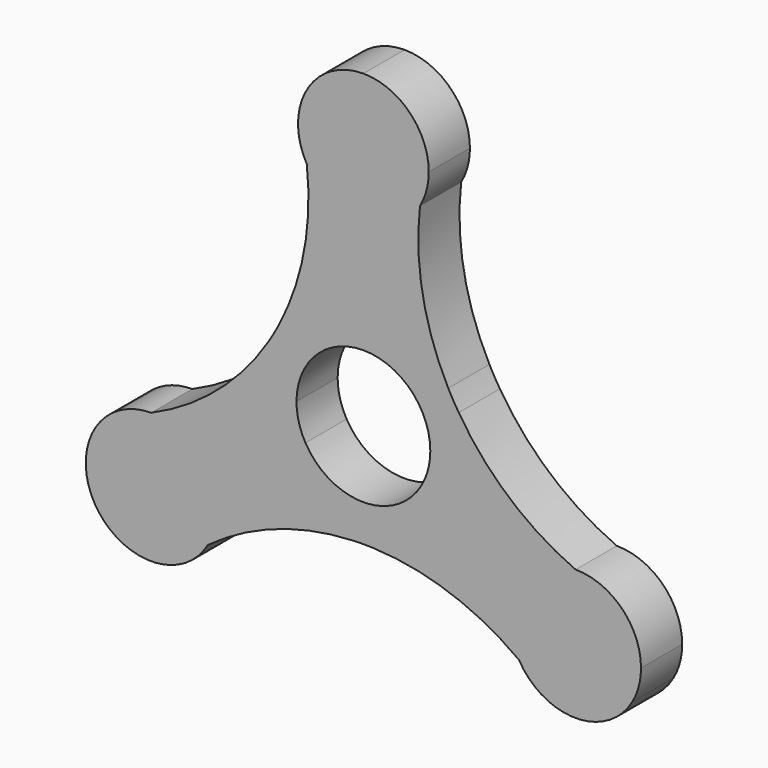
from build123d import *

# Parameters (mm, degrees)
F1_DEPTH = 5


# Not quite as in the source:
# - a feature names something its author has since deleted; it is built from what else it names


with BuildPart() as f1:
    # F0 (on Front) → F1 (new body)
    with BuildSketch(Plane.XZ):
        with BuildLine():
            ThreePointArc((-6.5, 0), (-4.5961940777, 4.5961940777), (0, 6.5))
            Line((0, 6.5), (0, 10.16))
            ThreePointArc((0, 10.16), (-4.6323577324, 9.0425030738), (-8.2456907547, 5.9358389447))
            ThreePointArc((-8.2456907547, 5.9358389447), (-8.7368966018, 5.0442496049), (-9.2634326962, 4.173058193))
            ThreePointArc((-9.2634326962, 4.173058193), (-9.9333296581, 2.1341419594), (-10.16, 0))
            Line((-10.16, 0), (-6.5, 0))
        make_face()
        with BuildLine():
            ThreePointArc((-5.6291651246, -3.25), (-6.2785178709, -1.6823237932), (-6.5, 0))
            Line((-6.5, 0), (-10.16, 0))
            ThreePointArc((-10.16, 0), (-9.8138063951, -2.6296014982), (-8.7988181024, -5.08))
            Line((-8.7988181024, -5.08), (-5.6291651246, -3.25))
        make_face()
        with BuildLine():
            ThreePointArc((-1.0177419415, -10.1088971377), (-0.508973166, -10.0935992038), (0, -10.0884992098))
            Line((0, -10.0884992098), (0, -6.5))
            ThreePointArc((0, -6.5), (-3.25, -5.6291651246), (-5.6291651246, -3.25))
            Line((-5.6291651246, -3.25), (-8.7988181024, -5.08))
            ThreePointArc((-8.7988181024, -5.08), (-5.5148585095, -8.5329910126), (-1.0177419415, -10.1088971377))
        make_face()
        with BuildLine():
            ThreePointArc((1.0177419415, -10.1088971377), (5.5148585095, -8.5329910126), (8.7988181024, -5.08))
            Line((8.7988181024, -5.08), (5.6291651246, -3.25))
            ThreePointArc((5.6291651246, -3.25), (3.25, -5.6291651246), (0, -6.5))
            Line((0, -6.5), (0, -10.0884992098))
            ThreePointArc((0, -10.0884992098), (0.508973166, -10.0935992038), (1.0177419415, -10.1088971377))
        make_face()
        with BuildLine():
            ThreePointArc((8.7988181024, -5.08), (9.8138063951, -2.6296014982), (10.16, 0))
            Line((10.16, 0), (6.5, 0))
            ThreePointArc((6.5, 0), (6.2785178709, -1.6823237932), (5.6291651246, -3.25))
            Line((5.6291651246, -3.25), (8.7988181024, -5.08))
        make_face()
        with BuildLine():
            Line((6.5, 0), (10.16, 0))
            ThreePointArc((10.16, 0), (9.9333296581, 2.1341419594), (9.2634326962, 4.173058193))
            ThreePointArc((9.2634326962, 4.173058193), (8.7368966018, 5.0442496049), (8.2456907547, 5.9358389447))
            ThreePointArc((8.2456907547, 5.9358389447), (4.6323577324, 9.0425030738), (0, 10.16))
            Line((0, 10.16), (0, 6.5))
            ThreePointArc((0, 6.5), (4.5961940777, 4.5961940777), (6.5, 0))
        make_face()
        with BuildLine():
            ThreePointArc((-8.2456907547, 5.9358389447), (-4.6323577324, 9.0425030738), (0, 10.16))
            Line((0, 10.16), (0, 15.875))
            Line((0, 15.875), (0, 17.4625))
            ThreePointArc((0, 17.4625), (-3.175, 18.313238686), (-5.499261314, 20.6375))
            ThreePointArc((-5.499261314, 20.6375), (-5.7658770412, 13.0799448007), (-8.2456907547, 5.9358389447))
        make_face()
        with BuildLine():
            Line((-5.499261314, 20.6375), (0, 23.8125))
            Line((0, 23.8125), (0, 30.1625))
            ThreePointArc((0, 30.1625), (-5.499261314, 26.9875), (-5.499261314, 20.6375))
        make_face()
        with BuildLine():
            Line((0, 23.8125), (5.499261314, 20.6375))
            ThreePointArc((5.499261314, 20.6375), (6.1336289969, 22.1689990636), (6.35, 23.8125))
            ThreePointArc((6.35, 23.8125), (4.4901280605, 28.3026280605), (0, 30.1625))
            Line((0, 30.1625), (0, 23.8125))
        make_face()
        with BuildLine():
            ThreePointArc((0, 17.4625), (3.175, 18.313238686), (5.499261314, 20.6375))
            Line((5.499261314, 20.6375), (0, 23.8125))
            Line((0, 23.8125), (0, 17.4625))
        make_face()
        with BuildLine():
            ThreePointArc((-5.499261314, 20.6375), (-3.175, 18.313238686), (0, 17.4625))
            Line((0, 17.4625), (0, 23.8125))
            Line((0, 23.8125), (-5.499261314, 20.6375))
        make_face()
        with BuildLine():
            Line((-20.6222299276, -5.55625), (-20.6222299276, -11.90625))
            Line((-20.6222299276, -11.90625), (-15.1229686136, -8.73125))
            ThreePointArc((-15.1229686136, -8.73125), (-17.4472299276, -6.406988686), (-20.6222299276, -5.55625))
        make_face()
        with BuildLine():
            Line((-23.7972299276, -6.406988686), (-20.6222299276, -11.90625))
            Line((-20.6222299276, -11.90625), (-20.6222299276, -5.55625))
            ThreePointArc((-20.6222299276, -5.55625), (-22.265730864, -5.7726210031), (-23.7972299276, -6.406988686))
        make_face()
        with BuildLine():
            ThreePointArc((-23.7972299276, -6.406988686), (-26.7558589246, -10.2627490636), (-26.1214912416, -15.08125))
            Line((-26.1214912416, -15.08125), (-20.6222299276, -11.90625))
            Line((-20.6222299276, -11.90625), (-23.7972299276, -6.406988686))
        make_face()
        with BuildLine():
            ThreePointArc((-26.1214912416, -15.08125), (-20.6222299276, -18.25625), (-15.1229686136, -15.08125))
            Line((-15.1229686136, -15.08125), (-20.6222299276, -11.90625))
            Line((-20.6222299276, -11.90625), (-26.1214912416, -15.08125))
        make_face()
        with BuildLine():
            Line((-20.6222299276, -11.90625), (-15.1229686136, -15.08125))
            ThreePointArc((-15.1229686136, -15.08125), (-14.4886009307, -13.5497509364), (-14.2722299276, -11.90625))
            ThreePointArc((-14.2722299276, -11.90625), (-14.4886009307, -10.2627490636), (-15.1229686136, -8.73125))
            Line((-15.1229686136, -8.73125), (-20.6222299276, -11.90625))
        make_face()
        with BuildLine():
            Line((20.6222299276, -11.90625), (15.1229686136, -15.08125))
            ThreePointArc((15.1229686136, -15.08125), (20.6222299276, -18.25625), (26.1214912416, -15.08125))
            Line((26.1214912416, -15.08125), (20.6222299276, -11.90625))
        make_face()
        with BuildLine():
            ThreePointArc((26.9722299276, -11.90625), (25.1123579882, -7.4161219395), (20.6222299276, -5.55625))
            Line((20.6222299276, -5.55625), (20.6222299276, -11.90625))
            Line((20.6222299276, -11.90625), (26.1214912416, -15.08125))
            ThreePointArc((26.1214912416, -15.08125), (26.7558589246, -13.5497509364), (26.9722299276, -11.90625))
        make_face()
        with BuildLine():
            Line((20.6222299276, -11.90625), (20.6222299276, -5.55625))
            ThreePointArc((20.6222299276, -5.55625), (17.4472299276, -6.406988686), (15.1229686136, -8.73125))
            Line((15.1229686136, -8.73125), (20.6222299276, -11.90625))
        make_face()
        with BuildLine():
            ThreePointArc((15.1229686136, -8.73125), (14.2722299276, -11.90625), (15.1229686136, -15.08125))
            Line((15.1229686136, -15.08125), (20.6222299276, -11.90625))
            Line((20.6222299276, -11.90625), (15.1229686136, -8.73125))
        make_face()
        with BuildLine():
            ThreePointArc((-15.1229686136, -15.08125), (-8.4446259569, -11.5333683931), (-1.0177419415, -10.1088971377))
            ThreePointArc((-1.0177419415, -10.1088971377), (-5.5148585095, -8.5329910126), (-8.7988181024, -5.08))
            Line((-8.7988181024, -5.08), (-13.7481532851, -7.9375))
            Line((-13.7481532851, -7.9375), (-15.1229686136, -8.73125))
            ThreePointArc((-15.1229686136, -8.73125), (-14.4886009307, -10.2627490636), (-14.2722299276, -11.90625))
            ThreePointArc((-14.2722299276, -11.90625), (-14.4886009307, -13.5497509364), (-15.1229686136, -15.08125))
        make_face()
        with BuildLine():
            ThreePointArc((0, 10.16), (4.6323577324, 9.0425030738), (8.2456907547, 5.9358389447))
            ThreePointArc((8.2456907547, 5.9358389447), (5.7658770412, 13.0799448007), (5.499261314, 20.6375))
            ThreePointArc((5.499261314, 20.6375), (3.175, 18.313238686), (0, 17.4625))
            Line((0, 17.4625), (0, 15.875))
            Line((0, 15.875), (0, 10.16))
        make_face()
        with BuildLine():
            Line((12.5597401985, 0), (10.16, 0))
            ThreePointArc((10.16, 0), (9.8138063951, -2.6296014982), (8.7988181024, -5.08))
            Line((8.7988181024, -5.08), (13.7481532851, -7.9375))
            Line((13.7481532851, -7.9375), (15.1229686136, -8.73125))
            ThreePointArc((15.1229686136, -8.73125), (17.4472299276, -6.406988686), (20.6222299276, -5.55625))
            ThreePointArc((20.6222299276, -5.55625), (16.3207116364, -3.1703097876), (12.5597401985, 0))
        make_face()
        with BuildLine():
            ThreePointArc((-8.7988181024, -5.08), (-9.8138063951, -2.6296014982), (-10.16, 0))
            Line((-10.16, 0), (-12.5597401985, 0))
            ThreePointArc((-12.5597401985, 0), (-16.3207116364, -3.1703097876), (-20.6222299276, -5.55625))
            ThreePointArc((-20.6222299276, -5.55625), (-17.4472299276, -6.406988686), (-15.1229686136, -8.73125))
            Line((-15.1229686136, -8.73125), (-13.7481532851, -7.9375))
            Line((-13.7481532851, -7.9375), (-8.7988181024, -5.08))
        make_face()
        with BuildLine():
            Line((13.7481532851, -7.9375), (8.7988181024, -5.08))
            ThreePointArc((8.7988181024, -5.08), (5.5148585095, -8.5329910126), (1.0177419415, -10.1088971377))
            ThreePointArc((1.0177419415, -10.1088971377), (8.4446259569, -11.5333683931), (15.1229686136, -15.08125))
            ThreePointArc((15.1229686136, -15.08125), (14.2722299276, -11.90625), (15.1229686136, -8.73125))
            Line((15.1229686136, -8.73125), (13.7481532851, -7.9375))
        make_face()
        with BuildLine():
            Line((-12.5597401985, 0), (-10.16, 0))
            ThreePointArc((-10.16, 0), (-9.9333296581, 2.1341419594), (-9.2634326962, 4.173058193))
            ThreePointArc((-9.2634326962, 4.173058193), (-10.8020734635, 2.0000245587), (-12.5597401985, 0))
        make_face()
        with BuildLine():
            ThreePointArc((9.2634326962, 4.173058193), (9.9333296581, 2.1341419594), (10.16, 0))
            Line((10.16, 0), (12.5597401985, 0))
            ThreePointArc((12.5597401985, 0), (10.8020734635, 2.0000245587), (9.2634326962, 4.173058193))
        make_face()
    extrude(amount=F1_DEPTH)


solid = f1.part
